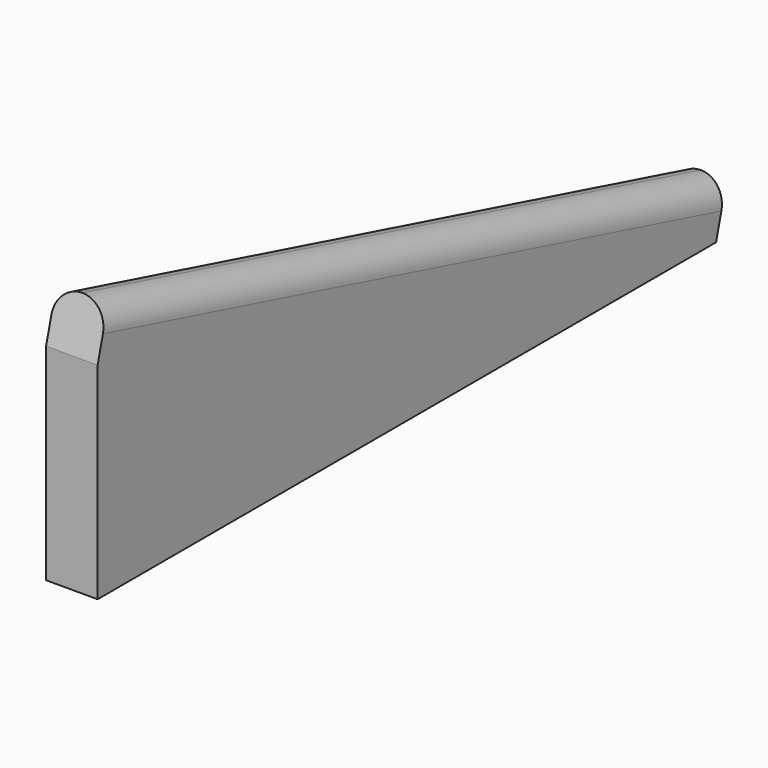
from build123d import *

# Parameters (mm, degrees)
F1_DEPTH = 10
F2_R     = 4.99999


# Not quite as in the source:
# - a fillet or chamfer is up to 0.001 mm smaller than in the source, because OpenCascade refuses the exact size


with BuildPart() as f1:
    # F0 (on Right) → F1 (new body)
    with BuildSketch(Plane.YZ):
        Polygon((0, 40), (0, 0), (150, 0), align=None)
        Polygon((2.5766265056, 49.662349396), (0, 40), (150, 0), (152.5766265056, 9.662349396), align=None)
    extrude(amount=F1_DEPTH)

    # F2 (radius 5 in the source; OpenCascade refuses exactly that, so slightly less here)
    f2_edges = [f1.edges().sort_by_distance(p)[0] for p in [
        (0, 77.576627, 29.662349),
        (10, 77.576627, 29.662349),
    ]]
    fillet(f2_edges, radius=F2_R)


solid = f1.part
